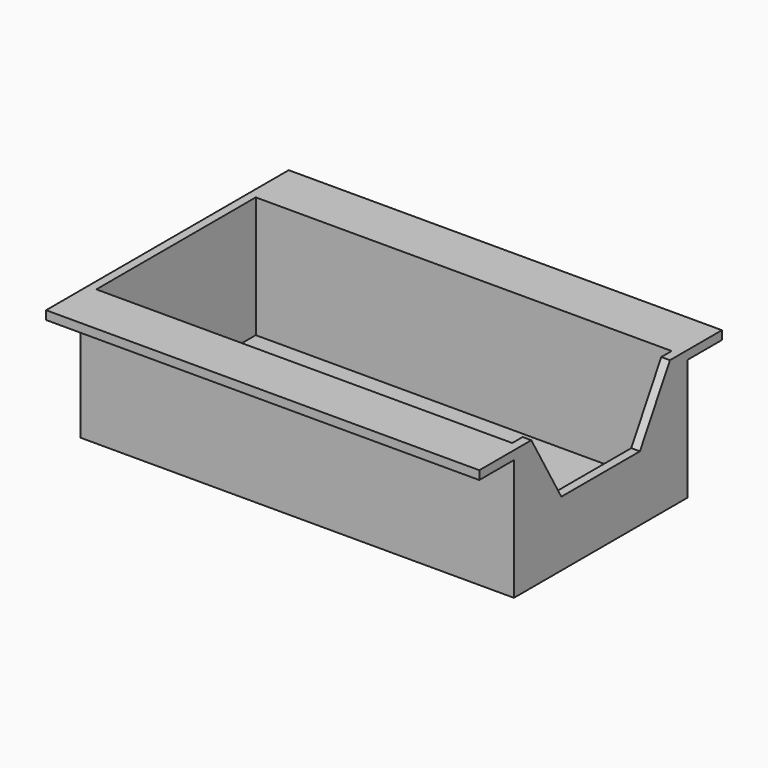
from build123d import *

# Parameters (mm, degrees)
F0_W     = 100
F0_H     = 50
F1_DEPTH = 30
F2_T     = -2
F3_W     = 100
F3_H     = 2
F4_DEPTH = 10
F7_DEPTH = 2


# Not quite as in the source:
# - a pattern or mirror of a feature is missing from the dataset's text; its kind, count and spacing are read off the source's solid


with BuildPart() as f1:
    # F0 (on Top) → F1 (new body)
    with BuildSketch(Plane.XY):
        Rectangle(F0_W, F0_H)
    extrude(amount=F1_DEPTH)

    # F2
    f2_openings = [f1.faces().sort_by_distance(p)[0] for p in [
        (0, 0, 30),
    ]]
    offset(amount=F2_T, openings=f2_openings)

    # F3 (on face) → F4 (join)
    with BuildSketch(Plane(origin=(0, 25, 0), x_dir=(-1, 0, 0), z_dir=(0, 1, 0))):
        with Locations((0, 29)):
            Rectangle(F3_W, F3_H)
    f4 = extrude(amount=F4_DEPTH)

    # F4_copies: F4 across plane
    add(f4.mirror(Plane(origin=(0, 0, 0), x_dir=(0, 0, -1), z_dir=(0, -1, 0))))

    # F6 (on face) → F7 (cut, through all)
    with BuildSketch(Plane.YZ.offset(50)):
        Polygon((11.3397459622, 15), (20, 30), (-20, 30), (-11.3397459622, 15), align=None)
    extrude(amount=-F7_DEPTH, mode=Mode.SUBTRACT)


solid = f1.part
